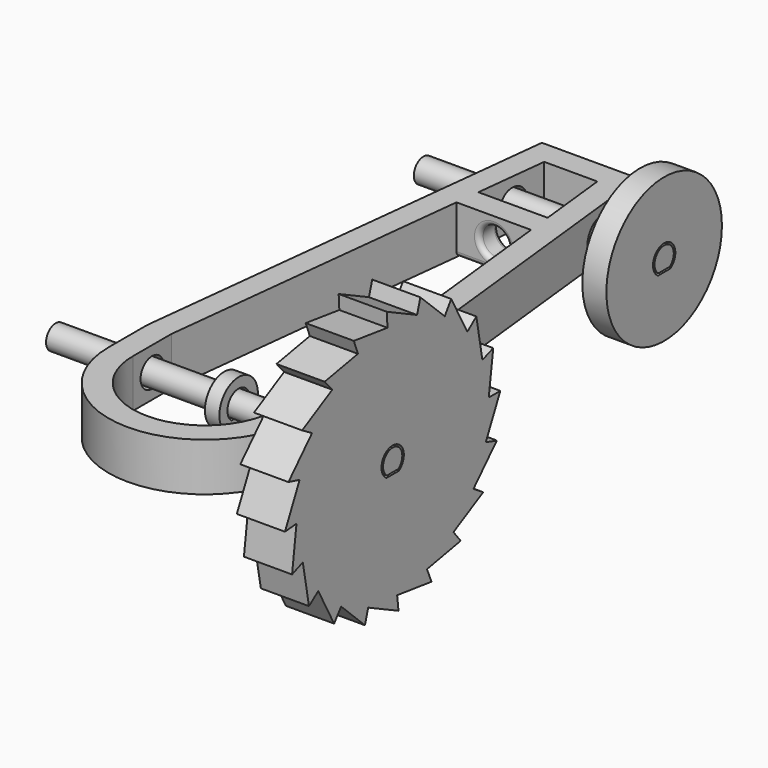
from build123d import *
from build123d import SkipClean  # not in build123d's __all__

# Parameters (mm, degrees)
F0_W           = 5.0307695212
F0_H           = 10
F1_DEPTH       = 10
F2_R           = 3
F3_DEPTH       = 25
F3_DEPTH_BACK  = 25
F4_R           = 3
F5_DEPTH       = 6
F6_R           = 0.99999
F7_DEPTH       = 25
F7_DEPTH_BACK  = 25
F8_DEPTH       = 35
F8_DEPTH_BACK  = 35
F10_R          = 5
F11_DEPTH      = 13
F10_R_2        = 15
F12_DEPTH      = 5
F13_DEPTH      = 4
F14_DEPTH      = 10
F15_R          = 2
F15_2_R        = 2
F2_R_2         = 5
F16_DEPTH      = 3
F17_R          = 1.5
F18_DEPTH      = 1
F18_DEPTH_BACK = 3


# Not quite as in the source:
# - a fillet or chamfer is up to 0.001 mm smaller than in the source, because OpenCascade refuses the exact size


with BuildPart() as f1:
    # F0 (on Top) → F1 (new body)
    with BuildSketch(Plane.XY):
        with Locations((-17.4846152394, -39.1540901363)):
            Rectangle(F0_W, F0_H)
        with Locations((17.4846152394, -39.1540901363)):
            Rectangle(F0_W, F0_H)
        Polygon((10, 55.8459098637), (-10, 55.8459098637), (-10, 50.8459098637), (-5.5247860344, 50.8459098637), (5.5247860344, 50.8459098637), (10, 50.8459098637), align=None)
        Polygon((7.7470082566, 30.8459098637), (14.9692304788, -34.1540901363), (20, -34.1540901363), (10, 55.8459098637), (10, 50.8459098637), (5.5247860344, 50.8459098637), (7.191452701, 35.8459098637), (7.7470082566, 35.8459098637), align=None)
        Polygon((-10, 55.8459098637), (-20, -34.1540901363), (-14.9692304788, -34.1540901363), (-7.7470082566, 30.8459098637), (-7.7470082566, 35.8459098637), (-7.191452701, 35.8459098637), (-5.5247860344, 50.8459098637), (-10, 50.8459098637), align=None)
        Polygon((-7.191452701, 35.8459098637), (-7.7470082566, 30.8459098637), (7.7470082566, 30.8459098637), (7.191452701, 35.8459098637), align=None)
        Polygon((-7.7470082566, 35.8459098637), (-7.7470082566, 30.8459098637), (-7.191452701, 35.8459098637), align=None)
        Polygon((7.191452701, 35.8459098637), (7.7470082566, 30.8459098637), (7.7470082566, 35.8459098637), align=None)
        with BuildLine():
            Line((-14.9692304788, -44.1540901363), (-20, -44.1540901363))
            ThreePointArc((-20, -44.1540901363), (0, -64.1540901363), (20, -44.1540901363))
            Line((20, -44.1540901363), (14.9692304788, -44.1540901363))
            ThreePointArc((14.9692304788, -44.1540901363), (0, -59.1233206151), (-14.9692304788, -44.1540901363))
        make_face()
    extrude(amount=F1_DEPTH)

    # F2 (on Right) → F3 (cut, two sides)
    with BuildSketch(Plane.YZ) as f3_sk:
        with Locations((-39.1540901363, 5)):
            Circle(F2_R)
        with BuildLine():
            ThreePointArc((-37.2646457735, 2.8), (-39.1540901363, 2.1), (-41.0435344991, 2.8))
            ThreePointArc((-41.0435344991, 2.8), (-40.3645882462, 7.6352787947), (-36.2540901363, 5))
            ThreePointArc((-36.2540901363, 5), (-36.5188113415, 3.7895018901), (-37.2646457735, 2.8))
        make_face(mode=Mode.SUBTRACT)
        with Locations((43.8459098637, 5)):
            Circle(F2_R)
        with BuildLine():
            ThreePointArc((42.3459098637, 3), (42.727875875, 7.2360679775), (46.3459098637, 5))
            ThreePointArc((46.3459098637, 5), (46.0819778412, 3.8819660113), (45.3459098637, 3))
            ThreePointArc((45.3459098637, 3), (43.8459098637, 2.5), (42.3459098637, 3))
        make_face(mode=Mode.SUBTRACT)
        with BuildLine():
            ThreePointArc((-37.6540901363, 3), (-36.9180221588, 3.8819660113), (-36.6540901363, 5))
            ThreePointArc((-36.6540901363, 5), (-40.272124125, 7.2360679775), (-40.6540901363, 3))
            Line((-40.6540901363, 3), (-37.6540901363, 3))
        make_face()
        with BuildLine():
            ThreePointArc((45.3459098637, 3), (46.0819778412, 3.8819660113), (46.3459098637, 5))
            ThreePointArc((46.3459098637, 5), (42.727875875, 7.2360679775), (42.3459098637, 3))
            Line((42.3459098637, 3), (45.3459098637, 3))
        make_face()
        with BuildLine():
            Line((45.3459098637, 3), (42.3459098637, 3))
            ThreePointArc((42.3459098637, 3), (43.8459098637, 2.5), (45.3459098637, 3))
        make_face()
        with BuildLine():
            ThreePointArc((-40.6540901363, 3), (-40.272124125, 7.2360679775), (-36.6540901363, 5))
            ThreePointArc((-36.6540901363, 5), (-36.9180221588, 3.8819660113), (-37.6540901363, 3))
            ThreePointArc((-37.6540901363, 3), (-37.8066571485, 2.8941927098), (-37.9666559276, 2.8))
            Line((-37.9666559276, 2.8), (-37.2646457735, 2.8))
            ThreePointArc((-37.2646457735, 2.8), (-36.5188113415, 3.7895018901), (-36.2540901363, 5))
            ThreePointArc((-36.2540901363, 5), (-40.3645882462, 7.6352787947), (-41.0435344991, 2.8))
            Line((-41.0435344991, 2.8), (-40.341524345, 2.8))
            ThreePointArc((-40.341524345, 2.8), (-40.5015231241, 2.8941927098), (-40.6540901363, 3))
        make_face()
        with BuildLine():
            Line((-37.6540901363, 3), (-40.6540901363, 3))
            ThreePointArc((-40.6540901363, 3), (-40.5015231241, 2.8941927098), (-40.341524345, 2.8))
            Line((-40.341524345, 2.8), (-37.9666559276, 2.8))
            ThreePointArc((-37.9666559276, 2.8), (-37.8066571485, 2.8941927098), (-37.6540901363, 3))
        make_face()
        with BuildLine():
            ThreePointArc((-37.9666559276, 2.8), (-39.1540901363, 2.5), (-40.341524345, 2.8))
            Line((-40.341524345, 2.8), (-41.0435344991, 2.8))
            ThreePointArc((-41.0435344991, 2.8), (-39.1540901363, 2.1), (-37.2646457735, 2.8))
            Line((-37.2646457735, 2.8), (-37.9666559276, 2.8))
        make_face()
        with BuildLine():
            Line((-37.9666559276, 2.8), (-40.341524345, 2.8))
            ThreePointArc((-40.341524345, 2.8), (-39.1540901363, 2.5), (-37.9666559276, 2.8))
        make_face()
    extrude(amount=-F3_DEPTH, mode=Mode.SUBTRACT)
    extrude(f3_sk.sketch, amount=F3_DEPTH_BACK, mode=Mode.SUBTRACT)

    # F4 (on face) → F5 (cut)
    with BuildSketch(Plane.XZ.offset(-30.8459098637)):
        with Locations((0, 5)):
            Circle(F4_R)
    extrude(amount=-F5_DEPTH, mode=Mode.SUBTRACT)

    # F6 (radius 1 in the source; OpenCascade refuses exactly that, so slightly less here)
    f6_edges = [f1.edges().sort_by_distance(p)[0] for p in [
        (-3, 30.84591, 5),
        (-3, 35.84591, 5),
        (0, 35.84591, 0),
        (0, 30.84591, 0),
    ]]
    fillet(f6_edges, radius=F6_R)


with BuildPart() as f7:
    # F2 (on Right) → F7 (new body, two sides)
    with BuildSketch(Plane.YZ) as f7_sk:
        with BuildLine():
            ThreePointArc((45.3459098637, 3), (46.0819778412, 3.8819660113), (46.3459098637, 5))
            ThreePointArc((46.3459098637, 5), (42.727875875, 7.2360679775), (42.3459098637, 3))
            Line((42.3459098637, 3), (45.3459098637, 3))
        make_face()
    extrude(amount=F7_DEPTH)
    extrude(f7_sk.sketch, amount=-F7_DEPTH_BACK)


with BuildPart() as f8:
    # F2 (on Right) → F8 (new body, two sides)
    with BuildSketch(Plane.YZ) as f8_sk:
        with BuildLine():
            ThreePointArc((-37.6540901363, 3), (-36.9180221588, 3.8819660113), (-36.6540901363, 5))
            ThreePointArc((-36.6540901363, 5), (-40.272124125, 7.2360679775), (-40.6540901363, 3))
            Line((-40.6540901363, 3), (-37.6540901363, 3))
        make_face()
    extrude(amount=F8_DEPTH)
    extrude(f8_sk.sketch, amount=-F8_DEPTH_BACK)


with BuildPart() as f11:
    # F10 (on offset) → F11 (new body)
    with BuildSketch(Plane.YZ.offset(25)):
        with Locations((43.8459098637, 5)):
            Circle(F10_R)
        with BuildLine():
            ThreePointArc((42.2180278041, 2.6), (42.4877600143, 7.5623093073), (46.7459098637, 5))
            ThreePointArc((46.7459098637, 5), (46.408219171, 3.6418501505), (45.4737919233, 2.6))
            ThreePointArc((45.4737919233, 2.6), (43.8459098637, 2.1), (42.2180278041, 2.6))
        make_face(mode=Mode.SUBTRACT)
        with BuildLine():
            Line((45.4737919233, 2.6), (42.2180278041, 2.6))
            ThreePointArc((42.2180278041, 2.6), (43.8459098637, 2.1), (45.4737919233, 2.6))
        make_face()
    extrude(amount=-F11_DEPTH)

    # F10 (on offset) → F12 (join)
    with BuildSketch(Plane.YZ.offset(25)):
        with Locations((43.8459098637, 5)):
            Circle(F10_R_2)
        with Locations((43.8459098637, 5)):
            Circle(F10_R, mode=Mode.SUBTRACT)
    extrude(amount=-F12_DEPTH)

    # F15
    f15_edges = [f11.edges().sort_by_distance(p)[0] for p in [
        (12, 38.84591, 5),
    ]]
    fillet(f15_edges, radius=F15_R)


with BuildPart() as f13:
    # F10 (on offset) → F13 (new body)
    with BuildSketch(Plane.YZ.offset(25)):
        with Locations((-39.1540901363, 5)):
            Circle(F10_R)
        with BuildLine():
            ThreePointArc((-40.7819721959, 2.6), (-40.5122399857, 7.5623093073), (-36.2540901363, 5))
            ThreePointArc((-36.2540901363, 5), (-36.591780829, 3.6418501505), (-37.5262080767, 2.6))
            ThreePointArc((-37.5262080767, 2.6), (-39.1540901363, 2.1), (-40.7819721959, 2.6))
        make_face(mode=Mode.SUBTRACT)
        with BuildLine():
            Line((-37.5262080767, 2.6), (-40.7819721959, 2.6))
            ThreePointArc((-40.7819721959, 2.6), (-39.1540901363, 2.1), (-37.5262080767, 2.6))
        make_face()
    extrude(amount=-F13_DEPTH)

    # F10 (on offset) → F14 (join)
    with BuildSketch(Plane.YZ.offset(25)):
        with BuildLine():
            ThreePointArc((-14.9766480513, -1.3601331924), (-14.3605823961, 1.7934482794), (-14.1540901363, 5))
            ThreePointArc((-14.1540901363, 5), (-14.1656080498, 5.7587904942), (-14.2001511774, 6.5168818137))
            ThreePointArc((-14.2001511774, 6.5168818137), (-14.7340955947, 10.3538646405), (-15.8544142437, 14.0622901797))
            ThreePointArc((-15.8544142437, 14.0622901797), (-17.5467124817, 17.5746264712), (-19.764515266, 20.7811402107))
            ThreePointArc((-19.764515266, 20.7811402107), (-22.4880569089, 23.6344663584), (-25.6264934276, 26.0238941989))
            ThreePointArc((-25.6264934276, 26.0238941989), (-29.0951104494, 27.887047159), (-32.8132327049, 29.182504565))
            ThreePointArc((-32.8132327049, 29.182504565), (-36.6270055915, 29.8719489325), (-40.5015101711, 29.9636627771))
            ThreePointArc((-40.5015101711, 29.9636627771), (-44.3993250567, 29.4435576508), (-48.1673646879, 28.3186809631))
            ThreePointArc((-48.1673646879, 28.3186809631), (-51.6534434584, 26.6510084414), (-54.8408601441, 24.4660023303))
            ThreePointArc((-54.8408601441, 24.4660023303), (-57.6909133357, 21.7745696121), (-60.085209418, 18.6707075755))
            ThreePointArc((-60.085209418, 18.6707075755), (-61.9896413023, 15.1753428908), (-63.3151669338, 11.4220221103))
            ThreePointArc((-63.3151669338, 11.4220221103), (-64.0168461692, 7.6159821196), (-64.1226827269, 3.7472494093))
            ThreePointArc((-64.1226827269, 3.7472494093), (-63.609495659, -0.1897148977), (-62.4795217853, -3.995790037))
            ThreePointArc((-62.4795217853, -3.995790037), (-60.752213979, -7.5905141466), (-58.475255219, -10.8648220868))
            ThreePointArc((-58.475255219, -10.8648220868), (-55.7135250048, -13.7292583098), (-52.5323204955, -16.1192554901))
            ThreePointArc((-52.5323204955, -16.1192554901), (-49.1436313044, -17.9174402421), (-45.5197214589, -19.175995075))
            ThreePointArc((-45.5197214589, -19.175995075), (-41.7828229709, -19.8614111362), (-37.9852146111, -19.9726596502))
            ThreePointArc((-37.9852146111, -19.9726596502), (-34.0462591754, -19.4726390664), (-30.2361468593, -18.3553053439))
            ThreePointArc((-30.2361468593, -18.3553053439), (-26.6405314571, -16.6428013247), (-23.3624825469, -14.3810507905))
            ThreePointArc((-23.3624825469, -14.3810507905), (-20.5325698167, -11.6804970246), (-18.1585535179, -8.5715674152))
            ThreePointArc((-18.1585535179, -8.5715674152), (-16.281602359, -5.0920415614), (-14.9766480513, -1.3601331924))
        make_face()
        with Locations((-39.1540901363, 5)):
            Circle(F10_R, mode=Mode.SUBTRACT)
        with Locations((-39.1540901363, 5)):
            Circle(F10_R)
        with BuildLine():
            ThreePointArc((-40.7819721959, 2.6), (-40.5122399857, 7.5623093073), (-36.2540901363, 5))
            ThreePointArc((-36.2540901363, 5), (-36.591780829, 3.6418501505), (-37.5262080767, 2.6))
            ThreePointArc((-37.5262080767, 2.6), (-39.1540901363, 2.1), (-40.7819721959, 2.6))
        make_face(mode=Mode.SUBTRACT)
        with BuildLine():
            Line((-37.5262080767, 2.6), (-40.7819721959, 2.6))
            ThreePointArc((-40.7819721959, 2.6), (-39.1540901363, 2.1), (-37.5262080767, 2.6))
        make_face()
        with BuildLine():
            ThreePointArc((-63.3151669338, 11.4220221103), (-61.9896413023, 15.1753428908), (-60.085209418, 18.6707075755))
            Line((-60.085209418, 18.6707075755), (-66.2133090863, 12.1971292759))
            Line((-66.2133090863, 12.1971292759), (-63.3151669338, 11.4220221103))
        make_face()
        with BuildLine():
            ThreePointArc((-60.085209418, 18.6707075755), (-57.6909133357, 21.7745696121), (-54.8408601441, 24.4660023303))
            Line((-54.8408601441, 24.4660023303), (-62.6649013876, 20.2066352065))
            Line((-62.6649013876, 20.2066352065), (-60.085209418, 18.6707075755))
        make_face()
        with BuildLine():
            ThreePointArc((-54.8408601441, 24.4660023303), (-51.6534434584, 26.6510084414), (-48.1673646879, 28.3186809631))
            Line((-48.1673646879, 28.3186809631), (-56.8150916742, 26.7276097323))
            Line((-56.8150916742, 26.7276097323), (-54.8408601441, 24.4660023303))
        make_face()
        with BuildLine():
            ThreePointArc((-48.1673646879, 28.3186809631), (-44.3993250567, 29.4435576508), (-40.5015101711, 29.9636627771))
            Line((-40.5015101711, 29.9636627771), (-49.2365000788, 31.1217344323))
            Line((-49.2365000788, 31.1217344323), (-48.1673646879, 28.3186809631))
        make_face()
        with BuildLine():
            ThreePointArc((-64.1226827269, 3.7472494093), (-64.0168461692, 7.6159821196), (-63.3151669338, 11.4220221103))
            Line((-63.3151669338, 11.4220221103), (-67.1129719015, 3.4831181863))
            Line((-67.1129719015, 3.4831181863), (-64.1226827269, 3.7472494093))
        make_face()
        with BuildLine():
            Line((-65.2758245686, -5.0824099425), (-62.4795217853, -3.995790037))
            ThreePointArc((-62.4795217853, -3.995790037), (-63.609495659, -0.1897148977), (-64.1226827269, 3.7472494093))
            Line((-64.1226827269, 3.7472494093), (-65.2758245686, -5.0824099425))
        make_face()
        with BuildLine():
            Line((-60.8816998686, -12.6610015379), (-58.475255219, -10.8648220868))
            ThreePointArc((-58.475255219, -10.8648220868), (-60.752213979, -7.5905141466), (-62.4795217853, -3.995790037))
            Line((-62.4795217853, -3.995790037), (-60.8816998686, -12.6610015379))
        make_face()
        with BuildLine():
            Line((-54.3607253428, -18.5108112513), (-52.5323204955, -16.1192554901))
            ThreePointArc((-52.5323204955, -16.1192554901), (-55.7135250048, -13.7292583098), (-58.475255219, -10.8648220868))
            Line((-58.475255219, -10.8648220868), (-54.3607253428, -18.5108112513))
        make_face()
        with BuildLine():
            Line((-46.3512194121, -22.05921895), (-45.5197214589, -19.175995075))
            ThreePointArc((-45.5197214589, -19.175995075), (-49.1436313044, -17.9174402421), (-52.5323204955, -16.1192554901))
            Line((-52.5323204955, -16.1192554901), (-46.3512194121, -22.05921895))
        make_face()
        with BuildLine():
            Line((-37.6372083226, -22.9588817653), (-37.9852146111, -19.9726596502))
            ThreePointArc((-37.9852146111, -19.9726596502), (-41.7828229709, -19.8614111362), (-45.5197214589, -19.175995075))
            Line((-45.5197214589, -19.175995075), (-37.6372083226, -22.9588817653))
        make_face()
        with BuildLine():
            Line((-29.0716801938, -21.1217344323), (-30.2361468593, -18.3553053439))
            ThreePointArc((-30.2361468593, -18.3553053439), (-34.0462591754, -19.4726390664), (-37.9852146111, -19.9726596502))
            Line((-37.9852146111, -19.9726596502), (-29.0716801938, -21.1217344323))
        make_face()
        with BuildLine():
            Line((-21.4930885984, -16.7276097323), (-23.3624825469, -14.3810507905))
            ThreePointArc((-23.3624825469, -14.3810507905), (-26.6405314571, -16.6428013247), (-30.2361468593, -18.3553053439))
            Line((-30.2361468593, -18.3553053439), (-21.4930885984, -16.7276097323))
        make_face()
        with BuildLine():
            Line((-15.6432788849, -10.2066352065), (-18.1585535179, -8.5715674152))
            ThreePointArc((-18.1585535179, -8.5715674152), (-20.5325698167, -11.6804970246), (-23.3624825469, -14.3810507905))
            Line((-23.3624825469, -14.3810507905), (-15.6432788849, -10.2066352065))
        make_face()
        with BuildLine():
            Line((-12.0948711862, -2.1971292759), (-14.9766480513, -1.3601331924))
            ThreePointArc((-14.9766480513, -1.3601331924), (-16.281602359, -5.0920415614), (-18.1585535179, -8.5715674152))
            Line((-18.1585535179, -8.5715674152), (-12.0948711862, -2.1971292759))
        make_face()
        with BuildLine():
            ThreePointArc((-14.2001511774, 6.5168818137), (-14.1656080498, 5.7587904942), (-14.1540901363, 5))
            ThreePointArc((-14.1540901363, 5), (-14.3605823961, 1.7934482794), (-14.9766480513, -1.3601331924))
            Line((-14.9766480513, -1.3601331924), (-11.195208371, 6.5168818137))
            Line((-11.195208371, 6.5168818137), (-14.2001511774, 6.5168818137))
        make_face()
        with BuildLine():
            ThreePointArc((-15.8544142437, 14.0622901797), (-14.7340955947, 10.3538646405), (-14.2001511774, 6.5168818137))
            Line((-14.2001511774, 6.5168818137), (-13.032355704, 15.0824099425))
            Line((-13.032355704, 15.0824099425), (-15.8544142437, 14.0622901797))
        make_face()
        with BuildLine():
            ThreePointArc((-19.764515266, 20.7811402107), (-17.5467124817, 17.5746264712), (-15.8544142437, 14.0622901797))
            Line((-15.8544142437, 14.0622901797), (-17.426480404, 22.6610015379))
            Line((-17.426480404, 22.6610015379), (-19.764515266, 20.7811402107))
        make_face()
        with BuildLine():
            ThreePointArc((-25.6264934276, 26.0238941989), (-22.4880569089, 23.6344663584), (-19.764515266, 20.7811402107))
            Line((-19.764515266, 20.7811402107), (-23.9474549298, 28.5108112513))
            Line((-23.9474549298, 28.5108112513), (-25.6264934276, 26.0238941989))
        make_face()
        with BuildLine():
            ThreePointArc((-32.8132327049, 29.182504565), (-29.0951104494, 27.887047159), (-25.6264934276, 26.0238941989))
            Line((-25.6264934276, 26.0238941989), (-31.9569608604, 32.05921895))
            Line((-31.9569608604, 32.05921895), (-32.8132327049, 29.182504565))
        make_face()
        with BuildLine():
            ThreePointArc((-40.5015101711, 29.9636627771), (-36.6270055915, 29.8719489325), (-32.8132327049, 29.182504565))
            Line((-32.8132327049, 29.182504565), (-40.6709719499, 32.9588817653))
            Line((-40.6709719499, 32.9588817653), (-40.5015101711, 29.9636627771))
        make_face()
    extrude(amount=F14_DEPTH)

    # F15#2
    f15_2_edges = [f13.edges().sort_by_distance(p)[0] for p in [
        (21, -44.15409, 5),
    ]]
    fillet(f15_2_edges, radius=F15_2_R)


with BuildPart() as f16:
    # F2 (on Right) → F16 (new body)
    with BuildSketch(Plane.YZ):
        with Locations((-39.1540901363, 5)):
            Circle(F2_R_2)
        with Locations((-39.1540901363, 5)):
            Circle(F2_R, mode=Mode.SUBTRACT)
        with Locations((-39.1540901363, 5)):
            Circle(F2_R)
        with BuildLine():
            ThreePointArc((-37.2646457735, 2.8), (-39.1540901363, 2.1), (-41.0435344991, 2.8))
            ThreePointArc((-41.0435344991, 2.8), (-40.3645882462, 7.6352787947), (-36.2540901363, 5))
            ThreePointArc((-36.2540901363, 5), (-36.5188113415, 3.7895018901), (-37.2646457735, 2.8))
        make_face(mode=Mode.SUBTRACT)
        with BuildLine():
            ThreePointArc((-37.9666559276, 2.8), (-39.1540901363, 2.5), (-40.341524345, 2.8))
            Line((-40.341524345, 2.8), (-41.0435344991, 2.8))
            ThreePointArc((-41.0435344991, 2.8), (-39.1540901363, 2.1), (-37.2646457735, 2.8))
            Line((-37.2646457735, 2.8), (-37.9666559276, 2.8))
        make_face()
        with BuildLine():
            Line((-37.9666559276, 2.8), (-40.341524345, 2.8))
            ThreePointArc((-40.341524345, 2.8), (-39.1540901363, 2.5), (-37.9666559276, 2.8))
        make_face()
    extrude(amount=F16_DEPTH)

    # F17 (on Top) → F18 (join, two sides)
    with BuildSketch(Plane.XY) as f18_sk:
        with Locations((1.5, -39.1540901363)):
            Circle(F17_R)
    with SkipClean():  # cleaning this boolean's faces spoils the solid; the shape is the same uncleaned
        extrude(amount=F18_DEPTH)
        extrude(f18_sk.sketch, amount=-F18_DEPTH_BACK)


solid = Compound([f1.part, f7.part, f8.part, f11.part, f13.part, f16.part])
